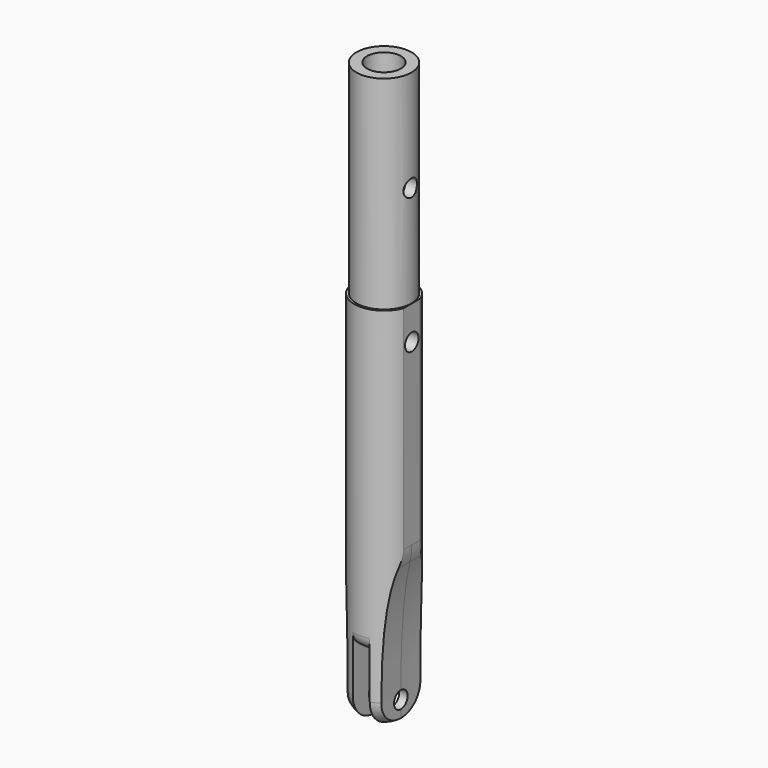
from build123d import *

# Parameters (mm, degrees)
F0_R           = 11.1125
F1_DEPTH       = 50.8
F2_R           = 11.1125
F3_DEPTH       = 88.9
F4_R           = 3.175
F5_DEPTH       = 11.1135
F5_DEPTH_BACK  = 11.1135
F6_W           = 12.7
F6_H           = 12.7
F7_DEPTH       = 11.1135001
F7_DEPTH_BACK  = 11.1135001
F8_R           = 3.175
F9_DEPTH       = 11.1135001
F9_DEPTH_BACK  = 11.1135001
F10_T2_ANGLE   = 331.6864704883
F10_T4_ANGLE   = 331.6864704883
F12_W          = 6.35
F12_H          = 31.75
F13_DEPTH      = 11.1135001
F13_DEPTH_BACK = 11.1135001
F14_R          = 5.08
F15_R          = 10.3124
F16_DEPTH      = 76.2
F17_R          = 3.175
F18_DEPTH      = 11.1135001
F18_DEPTH_BACK = 25.4
F11_R          = 6.35
F19_DEPTH      = 76.2
F19_DEPTH_BACK = 76.2010001
F20_W          = 15.9595024631
F20_H          = 158.0921553572
F21_DEPTH      = 25.4
F21_DEPTH_BACK = 25.4
F22_R          = 25.4


# Not quite as in the source:
# - a fillet or chamfer that OpenCascade refuses, or shapes differently, is made with other operations: its cross-section is extruded or revolved along the edge and cut away or added


with BuildPart() as f1:
    # F0 (on Top) → F1 (new body)
    with BuildSketch(Plane.XY):
        Circle(F0_R)
    extrude(amount=F1_DEPTH)

    # F2 (on face) → F3 (join)
    with BuildSketch(Plane(origin=(0, 0, 0), x_dir=(1, 0, 0), z_dir=(0, 0, -1))):
        Circle(F2_R)
    extrude(amount=F3_DEPTH)

    # F4 (on Right) → F5 (cut, two sides)
    with BuildSketch(Plane.YZ) as f5_sk:
        with Locations((0, 38.1)):
            Circle(F4_R)
    extrude(amount=-F5_DEPTH, mode=Mode.SUBTRACT)
    extrude(f5_sk.sketch, amount=F5_DEPTH_BACK, mode=Mode.SUBTRACT)

    # F6 (on Front) → F7 (cut, two sides)
    with BuildSketch(Plane.XZ) as f7_sk:
        with Locations((-12.7, -95.25)):
            Rectangle(F6_W, F6_H)
        with BuildLine():
            Line((-19.05, -88.9), (-6.35, -88.9))
            add(Edge.make_bspline(
                [(-12.7, -25.4), (-6.5615815111, -39.3321929336), (-6.1049603775, -64.6134701729), (-6.35, -88.9)],
                knots=[0, 0, 0, 0, 63.8167101941, 63.8167101941, 63.8167101941, 63.8167101941], degree=3))
            Line((-12.7, -25.4), (-19.05, -88.9))
        make_face()
        with BuildLine():
            add(Edge.make_bspline(
                [(12.7, -25.4), (6.5615815111, -39.3321929336), (6.1049603775, -64.6134701729), (6.35, -88.9)],
                knots=[0, 0, 0, 0, 63.8167101941, 63.8167101941, 63.8167101941, 63.8167101941], degree=3))
            Line((6.35, -88.9), (19.05, -88.9))
            Line((19.05, -88.9), (12.7, -25.4))
        make_face()
        with Locations((12.7, -95.25)):
            Rectangle(F6_W, F6_H)
    extrude(amount=-F7_DEPTH, mode=Mode.SUBTRACT)
    extrude(f7_sk.sketch, amount=F7_DEPTH_BACK, mode=Mode.SUBTRACT)

    # F8 (on Right) → F9 (cut, two sides)
    with BuildSketch(Plane.YZ) as f9_sk:
        with Locations((0, -81.28)):
            Circle(F8_R)
    extrude(amount=-F9_DEPTH, mode=Mode.SUBTRACT)
    extrude(f9_sk.sketch, amount=F9_DEPTH_BACK, mode=Mode.SUBTRACT)

    # F10: fillet of radius 10.16 on 2 edges, made by hand

    # F10_s1 → F10_t2 (revolve, cut)
    with BuildSketch(Plane(origin=(0, 0, 0), x_dir=(0, 0, 1), z_dir=(0.9696301822, -0.2445757752, 0))):
        with BuildLine():
            ThreePointArc((-78.74, 11.1125), (-85.9242048969, 8.1367048969), (-88.9, 0.9525))
            Line((-88.9, 0.9525), (-88.9, 11.1125))
            Line((-88.9, 11.1125), (-78.74, 11.1125))
        make_face()
    revolve(axis=Axis((0, 0, -88.9), (0, 0, -1)), revolution_arc=F10_T2_ANGLE, mode=Mode.SUBTRACT)

    # F10_s3 → F10_t4 (revolve, cut)
    with BuildSketch(Plane(origin=(0, 0, 0), x_dir=(0, 0, 1), z_dir=(-0.9696301822, 0.2445757752, 0))):
        with BuildLine():
            ThreePointArc((-78.74, 11.1125), (-85.9242048969, 8.1367048969), (-88.9, 0.9525))
            Line((-88.9, 0.9525), (-88.9, 11.1125))
            Line((-88.9, 11.1125), (-78.74, 11.1125))
        make_face()
    revolve(axis=Axis((0, 0, -88.9), (0, 0, -1)), revolution_arc=F10_T4_ANGLE, mode=Mode.SUBTRACT)

    # F12 (on Front) → F13 (cut, two sides)
    with BuildSketch(Plane.XZ) as f13_sk:
        with Locations((0, -78.74)):
            Rectangle(F12_W, F12_H)
    extrude(amount=-F13_DEPTH, mode=Mode.SUBTRACT)
    extrude(f13_sk.sketch, amount=F13_DEPTH_BACK, mode=Mode.SUBTRACT)

    # F14
    f14_edges = [f1.edges().sort_by_distance(p)[0] for p in [
        (0, 11.1125, -62.865),
        (0, -11.1125, -62.865),
    ]]
    fillet(f14_edges, radius=F14_R)

    # F15 (on face) → F16 (join)
    with BuildSketch(Plane.XY.offset(50.8)):
        Circle(F15_R)
    extrude(amount=F16_DEPTH)

    # F17 (on Right) → F18 (cut, two sides)
    with BuildSketch(Plane.YZ) as f18_sk:
        with Locations((0, 88.9)):
            Circle(F17_R)
    extrude(amount=F18_DEPTH, mode=Mode.SUBTRACT)
    extrude(f18_sk.sketch, amount=-F18_DEPTH_BACK, mode=Mode.SUBTRACT)

    # F11 (on face) → F19 (cut, two sides)
    with BuildSketch(Plane.XY.offset(50.8)) as f19_sk:
        Circle(F11_R)
    extrude(amount=-F19_DEPTH, mode=Mode.SUBTRACT)
    extrude(f19_sk.sketch, amount=F19_DEPTH_BACK, mode=Mode.SUBTRACT)

    # F20 (on Front) → F21 (cut, two sides)
    with BuildSketch(Plane.XZ) as f21_sk:
        with Locations((-18.3937512316, -22.505544275)):
            Rectangle(F20_W, F20_H)
        with Locations((18.3937512316, -22.505544275)):
            Rectangle(F20_W, F20_H)
    extrude(amount=-F21_DEPTH, mode=Mode.SUBTRACT)
    extrude(f21_sk.sketch, amount=F21_DEPTH_BACK, mode=Mode.SUBTRACT)

    # F22
    f22_edges = [f1.edges().sort_by_distance(p)[0] for p in [
        (-10.414, -1.938831, -31.988044),
        (10.414, -1.93883, -31.988044),
    ]]
    fillet(f22_edges, radius=F22_R)


solid = f1.part
